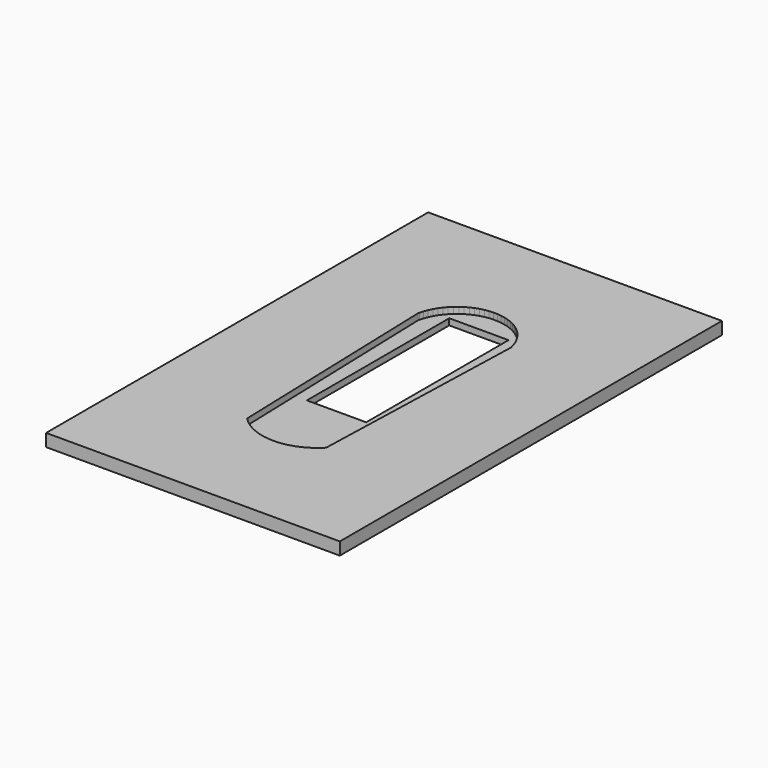
from build123d import *

# Parameters (mm, degrees)
F1_W     = 74.2999784
F1_H     = 120.793891
F2_DEPTH = 3.175
F3_DEPTH = 1.5748
F5_DEPTH = 1.6012
F7_DEPTH = 187


# Not quite as in the source:
# - an extrude ends at something that could not be found from the text; its depth is read off the source's solid


with BuildPart() as f2:
    # F1 (on Top) → F2 (new body)
    with BuildSketch(Plane.XY):
        with Locations((0, 44.9976621)):
            Rectangle(F1_W, F1_H)
    extrude(amount=-F2_DEPTH)

    # F0 (on Top) → F3 (cut)
    with BuildSketch(Plane.XY):
        Polygon((-11.67892, 70.7573642), (-11.7499892, 70.4366892), (-10.0000054, 14.202029), (-9.1080082, 13.367766), (-8.146669, 12.614402), (-7.1233538, 11.9477028), (-6.045835, 11.372723), (-4.9222914, 10.8938568), (-3.7612828, 10.514711), (-2.5716484, 10.2382066), (-1.3624306, 10.0664518), (-0.142875, 10.0007166), (1.0777982, 10.0415598), (2.2902418, 10.1886004), (3.4852864, 10.4407716), (4.653788, 10.7961176), (5.7868566, 11.2519714), (6.875907, 11.8048532), (7.9126334, 12.4505212), (8.889111, 13.1840986), (9.7979484, 13.9999974), (10.0000054, 14.202029), (11.7499892, 70.4366892), (11.4929158, 71.4514954), (11.1483648, 72.440038), (10.7189524, 73.3947986), (10.2079806, 74.3084874), (9.6193102, 75.1741702), (8.957437, 75.985243), (8.2274156, 76.735559), (7.4347324, 77.4193778), (6.5855088, 78.0315178), (5.6861456, 78.5673054), (4.7435008, 79.0226766), (3.7647626, 79.3941516), (2.7573732, 79.678911), (1.728978, 79.8747958), (0.687451, 79.980282), (-0.3593084, 79.9946076), (-1.40335, 79.917671), (-2.4366982, 79.7500056), (-3.4515044, 79.4929068), (-4.440047, 79.1483558), (-5.3947822, 78.7189688), (-6.3084964, 78.207997), (-7.1741538, 77.6193266), (-7.985252, 76.9574534), (-8.7355426, 76.2274066), (-9.4193614, 75.4347488), (-10.0315014, 74.5854998), (-10.5673144, 73.6861366), (-11.0226602, 72.7434918), (-11.3941352, 71.7647536), align=None)
    extrude(amount=-F3_DEPTH, mode=Mode.SUBTRACT)

    # F4 (on face) → F5 (cut, through all)
    with BuildSketch(Plane.XY.offset(-1.5748)):
        Polygon((7.5, 74.9946076), (-7.5, 74.9946076), (-7.5, 29.9946076), (0, 29.9946076), (7.5, 29.9946076), align=None)
    extrude(amount=-F5_DEPTH, mode=Mode.SUBTRACT)

    # F6 (on Top) → F7 (cut, through all)
    with BuildSketch(Plane.XY):
        Polygon((-10.7912024307, 73.8066075367), (-11.2561967507, 72.8439886266), (-11.6355402146, 71.8445191089), (-11.9253249204, 70.8194431888), (-12.0048558585, 70.4605875443), (-10.2505992593, 14.0886235531), (-9.2734099156, 13.1746824405), (-8.2946132005, 12.4076376674), (-7.2527155028, 11.7288318004), (-6.155627842, 11.1434097699), (-5.0116809128, 10.6558474546), (-3.8295896081, 10.2698167625), (-2.6183487878, 9.9882904244), (-1.3871727116, 9.8134167162), (-0.1454684467, 9.7464876822), (1.0973724592, 9.7880726041), (2.3318323641, 9.9377832588), (3.5485785618, 10.1945338008), (4.7383012319, 10.5563332129), (5.8919487163, 11.0204662668), (7.0007735223, 11.5833870046), (8.0563268906, 12.240780346), (9.0505396482, 12.9876812578), (9.9727120125, 13.8155513756), (10.250752791, 14.0935572024), (12.00497648, 70.4644636422), (11.7364147609, 71.5246203819), (11.3845631065, 72.5341091055), (10.9460529906, 73.5090976745), (10.4242555991, 74.442144141), (9.8231127621, 75.3261685703), (9.1472184874, 76.1544230786), (8.4017288342, 76.9206373493), (7.5922505458, 77.6189446578), (6.7250358763, 78.2440530365), (5.8066165367, 78.7911931616), (4.8440002256, 79.2562121642), (3.8445253314, 79.6355576688), (2.8157931282, 79.9263500525), (1.7656080971, 80.1263852965), (0.7020137501, 80.2341064847), (-0.3669184196, 80.2487355339), (-1.4330803845, 80.1701688593), (-2.4883265282, 79.9989504193), (-3.5246322079, 79.7364047759), (-4.5341166426, 79.3845546164), (-5.509078548, 78.9460707649), (-6.4421534102, 78.4242719991), (-7.3261519012, 77.8231291621), (-8.154434062, 77.1472334884), (-8.9206223557, 76.4017179349), (-9.6189282578, 75.5922672148), (-10.2440360096, 74.725027477), align=None)
    extrude(amount=F7_DEPTH, mode=Mode.SUBTRACT)


solid = f2.part
